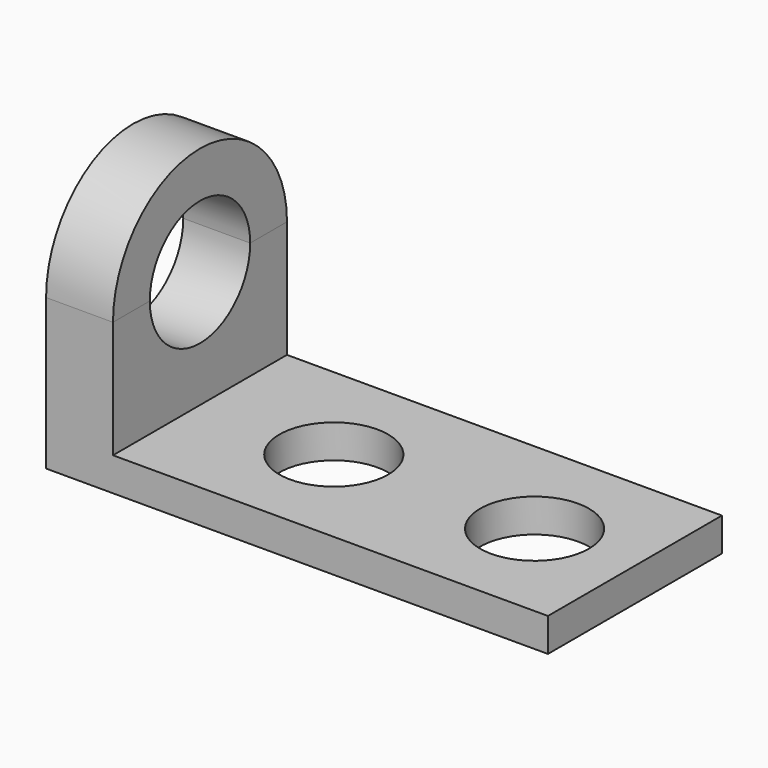
from build123d import *

# Parameters (mm, degrees)
F1_DEPTH = 82.55
F2_R     = 20.6375
F3_DEPTH = 12.701
F5_DEPTH = 25.4
F7_DEPTH = 25.401


# Not quite as in the source:
# - a feature of the source that left no trace in its solid (it failed there, or was rolled back) is left out


with BuildPart() as f1:
    # F0 (on Front) → F1 (new body)
    with BuildSketch(Plane.XZ):
        Polygon((0, 57.15), (0, 0), (190.5, 0), (190.5, 12.7), (25.4, 12.7), (25.4, 57.15), align=None)
    extrude(amount=F1_DEPTH)

    # F2 (on face) → F3 (cut, through all)
    with BuildSketch(Plane.XY.offset(12.7)):
        with Locations((76.2, -41.275)):
            Circle(F2_R)
        with Locations((152.4, -41.275)):
            Circle(F2_R)
    extrude(amount=-F3_DEPTH, mode=Mode.SUBTRACT)


with BuildPart() as f5:
    # F4 (on face) → F5 (new body)
    with BuildSketch(Plane.YZ.offset(25.4)):
        with BuildLine():
            Line((-82.55, 57.15), (0, 57.15))
            ThreePointArc((0, 57.15), (-41.275, 98.425), (-82.55, 57.15))
        make_face()
    extrude(amount=-F5_DEPTH)


with BuildPart() as f7_tool:
    # F6 (on face) → F7 (new body, through all)
    with BuildSketch(Plane.YZ.offset(25.4)):
        with BuildLine():
            Line((-65.0875, 57.15), (-17.4625, 57.15))
            ThreePointArc((-17.4625, 57.15), (-41.275, 80.9625), (-65.0875, 57.15))
        make_face()
        with BuildLine():
            ThreePointArc((-65.0875, 57.15), (-41.275, 33.3375), (-17.4625, 57.15))
            Line((-17.4625, 57.15), (-65.0875, 57.15))
        make_face()
    extrude(amount=-F7_DEPTH)


with BuildPart() as f1_1:
    add(f1.part)

    # F7: cut by f7_tool
    add(f7_tool.part, mode=Mode.SUBTRACT)


with BuildPart() as f5_1:
    add(f5.part)

    # F7: cut by f7_tool
    add(f7_tool.part, mode=Mode.SUBTRACT)


solid = Compound([f1_1.part, f5_1.part])
